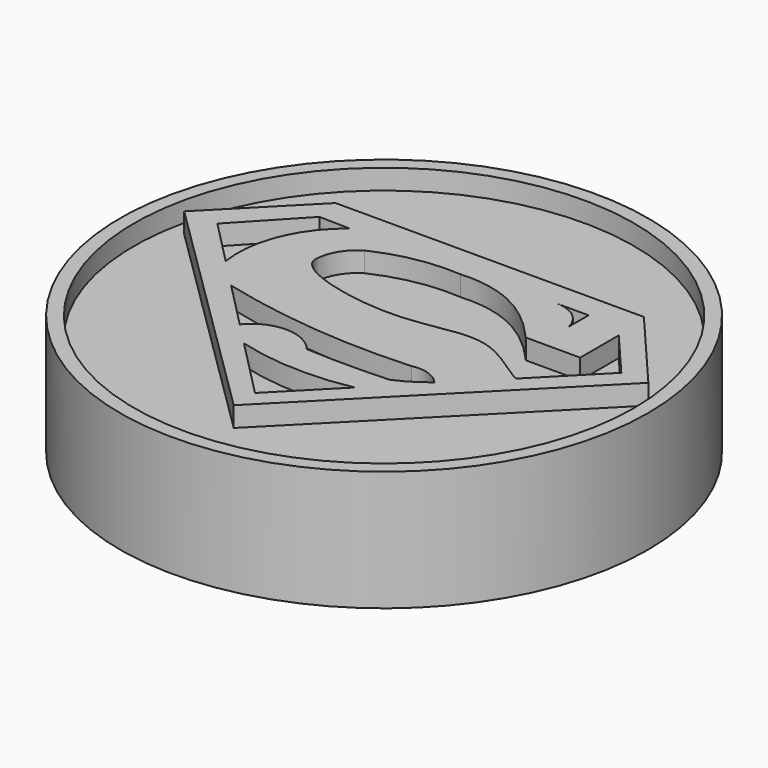
from build123d import *

# Parameters (mm, degrees)
F1_DEPTH = 60
F2_R     = 131.6532822565
F2_R_2   = 124.7334894873
F3_DEPTH = 60
F4_DEPTH = 50


with BuildPart() as f1:
    # F0 (on Top) → F1 (new body)
    with BuildSketch(Plane.XY):
        Polygon((74.9296570044, 62.355361724), (-78.8422822756, 62.355361724), (-120.5317750377, 20.0672930421), (-3.2890513343, -95.5764094054), (110.9969020086, 20.0672930421), align=None)
        with BuildLine():
            ThreePointArc((30.6225829023, -40.886171317), (10.024576741, -41.4386449004), (-10.5734294202, -40.886171317))
            ThreePointArc((-10.5734294202, -40.886171317), (-27.3146695696, -32.9122104229), (-44.055909719, -40.886171317))
            Line((-44.055909719, -40.886171317), (-67.174919563, -17.3738146812))
            ThreePointArc((-67.174919563, -17.3738146812), (-18.9151123365, -25.7248463855), (30.0547086439, -26.5647018575))
            ThreePointArc((30.0547086439, -26.5647018575), (38.5659779212, -26.967690046), (45.6699691909, -31.6727311968))
            ThreePointArc((45.6699691909, -31.6727311968), (38.4995277759, -36.8563818233), (30.6225829023, -40.886171317))
        make_face(mode=Mode.SUBTRACT)
        with BuildLine():
            Line((24.142164092, -54.4732124549), (-3.2890513343, -82.3466369568))
            Line((-3.2890513343, -82.3466369568), (-32.7572226476, -52.3770942299))
            ThreePointArc((-32.7572226476, -52.3770942299), (-4.428048629, -56.6966659367), (24.142164092, -54.4732124549))
        make_face(mode=Mode.SUBTRACT)
        with BuildLine():
            Line((-81.67515814, -2.6268690711), (-103.989661336, 20.0672930421))
            Line((-103.989661336, 20.0672930421), (-76.5038450393, 49.3119040818))
            Line((-76.5038450393, 49.3119040818), (-61.1454658014, 49.0162855328))
            ThreePointArc((-61.1454658014, 49.0162855328), (-78.4436240705, 25.9906593039), (-81.67515814, -2.6268690711))
        make_face(mode=Mode.SUBTRACT)
        with BuildLine():
            Line((76.9870403049, 20.0672930421), (76.9870403049, 44.1184047228))
            Line((76.9870403049, 44.1184047228), (97.5000919682, 20.0672930421))
            Line((97.5000919682, 20.0672930421), (69.0316228459, -8.8601063616))
            add(Edge.make_bspline(
                [(68.8241100173, -9.0709644323), (68.9152133704, -9.0266250767), (68.9840910354, -8.9558840502), (69.0316228459, -8.8601063616)],
                knots=[0.8556335845, 0.8556335845, 0.8556335845, 0.8556335845, 0.8617790869, 0.8617790869, 0.8617790869, 0.8617790869], degree=3))
            add(Edge.make_bspline(
                [(-55.3941001687, 20.0672930421), (-54.6137788828, 9.8420286504), (2.8320946288, -4.0014398965), (39.1107514545, 15.5059780363), (66.8637435516, -10.0250608833), (68.8241100173, -9.0709644323)],
                knots=[0.3747893908, 0.3747893908, 0.3747893908, 0.3747893908, 0.5560743676, 0.723394359, 0.8556335845, 0.8556335845, 0.8556335845, 0.8556335845], degree=3))
            add(Edge.make_bspline(
                [(-55.3453841257, 21.3418374189), (-55.4091134145, 20.912536879), (-55.4261568649, 20.4873612884), (-55.3941001687, 20.0672930421)],
                knots=[0.367341949, 0.367341949, 0.367341949, 0.367341949, 0.3747893908, 0.3747893908, 0.3747893908, 0.3747893908], degree=3))
            ThreePointArc((-55.3453841257, 21.3418374189), (-52.2632242925, 31.0147803908), (-45.0575761301, 38.1662955822))
            ThreePointArc((-45.0575761301, 38.1662955822), (-24.6682987221, 44.6929576974), (-3.2890513343, 45.8099772682))
            add(Edge.make_bspline(
                [(49.8549297409, 20.0672930421), (35.5399556775, 36.338533457), (19.7655314176, 47.3009599168), (-3.2890513343, 45.8099772682)],
                knots=[0, 0, 0, 0, 0.1881410109, 0.1881410109, 0.1881410109, 0.1881410109], degree=3))
            Line((49.8549297409, 20.0672930421), (76.9870403049, 20.0672930421))
        make_face(mode=Mode.SUBTRACT)
        with BuildLine():
            ThreePointArc((57.2370365458, 37.6215761842), (51.6712340933, 46.5316736156), (41.7582169371, 50.0101911218))
            Line((41.7582169371, 50.0101911218), (57.2370365458, 50.0101911218))
            Line((57.2370365458, 50.0101911218), (57.2370365458, 37.6215761842))
        make_face(mode=Mode.SUBTRACT)
        with BuildLine():
            add(Edge.make_bspline(
                [(68.8241100173, -9.0709644323), (68.9152133704, -9.0266250767), (68.9840910354, -8.9558840502), (69.0316228459, -8.8601063616)],
                knots=[0.8556335845, 0.8556335845, 0.8556335845, 0.8556335845, 0.8617790869, 0.8617790869, 0.8617790869, 0.8617790869], degree=3))
            Line((69.0316228459, -8.8601063616), (68.8241100173, -9.0709644323))
        make_face()
    extrude(amount=F1_DEPTH)


with BuildPart() as f3:
    # F2 (on Top) → F3 (new body)
    with BuildSketch(Plane.XY):
        with Locations((-4.7674374655, 0)):
            Circle(F2_R)
        with Locations((-4.7674374655, 0)):
            Circle(F2_R_2, mode=Mode.SUBTRACT)
    extrude(amount=F3_DEPTH)


with BuildPart() as f4:
    # F2 (on Top) → F4 (new body)
    with BuildSketch(Plane.XY):
        with Locations((-4.7674374655, 0)):
            Circle(F2_R_2)
    extrude(amount=F4_DEPTH)


solid = Compound([f1.part, f3.part, f4.part])
